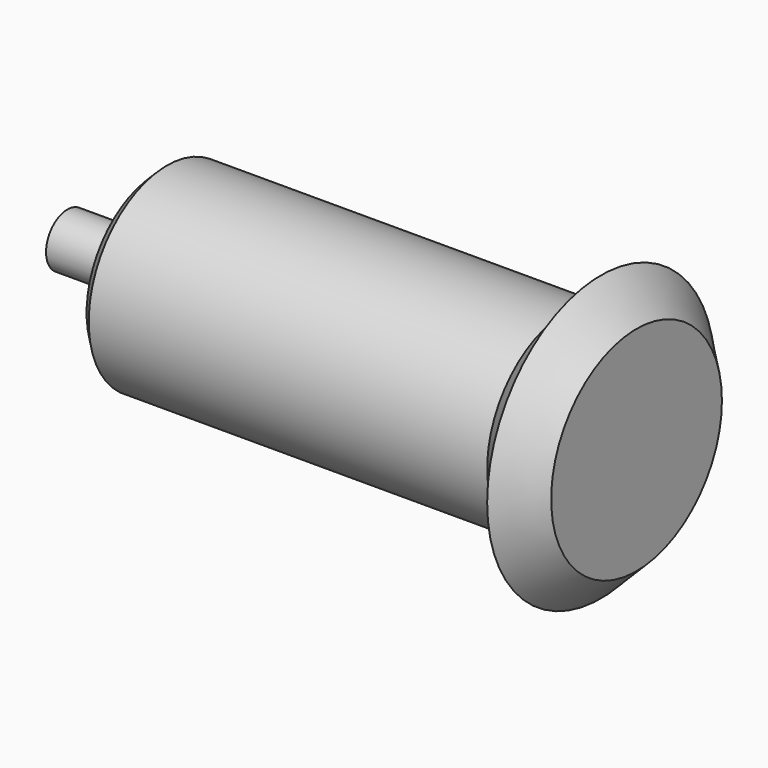
from build123d import *

# Parameters (mm, degrees)
F2_SIZE = 9.99999
F3_SIZE = 3


# Not quite as in the source:
# - a fillet or chamfer is up to 0.001 mm smaller than in the source, because OpenCascade refuses the exact size


with BuildPart() as f1:
    # F0 (on Top) → F1 (revolve)
    with BuildSketch(Plane.XY):
        Polygon((0, 7.5), (0, 0), (160, 0), (160, 40), (150, 40), (150, 27.5), (25, 27.5), (25, 7.5), align=None)
    revolve(axis=Axis((80, 0, 0), (-1, 0, 0)))

    # F2 (size 10 in the source; OpenCascade refuses exactly that, so slightly less here)
    f2_edges = [f1.edges().sort_by_distance(p)[0] for p in [
        (160, -40, 0),
        (150, -27.5, 0),
    ]]
    chamfer(f2_edges, length=F2_SIZE)

    # F3
    f3_edges = [f1.edges().sort_by_distance(p)[0] for p in [
        (25, -27.5, 0),
    ]]
    chamfer(f3_edges, length=F3_SIZE)


solid = f1.part
